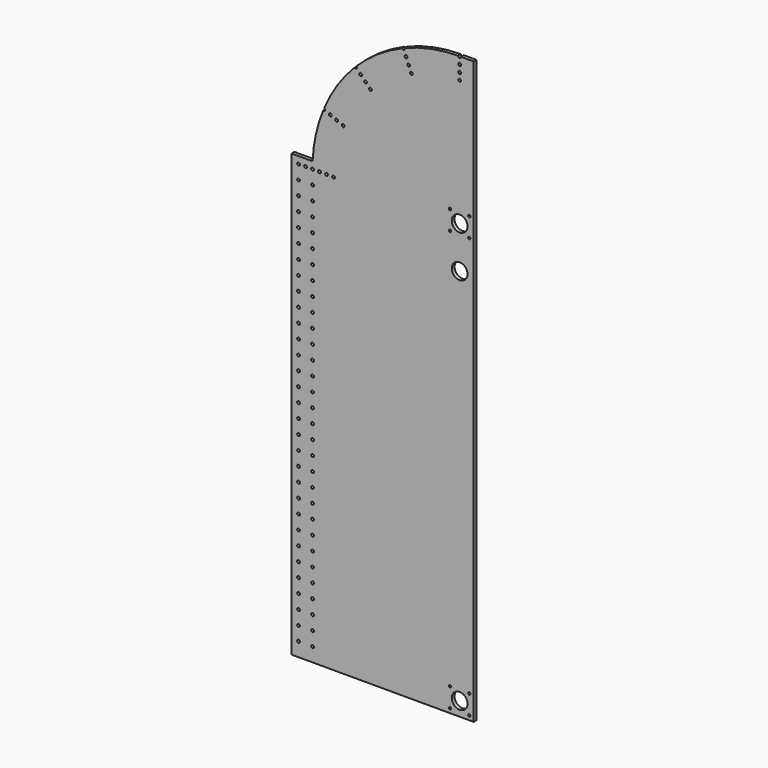
from build123d import *

# Parameters (mm, degrees)
F0_R     = 14.2875
F1_DEPTH = 6.35
F2_R     = 2.5527
F3_DEPTH = 25.4
F4_R     = 2.159
F5_DEPTH = 25.4
F7_D     = 5.1054
F9_DEPTH = 25.4


# Not quite as in the source:
# - a feature names something its author has since deleted; it is built from what else it names


with BuildPart() as f1:
    # F0 (on Front) → F1 (new body)
    with BuildSketch(Plane.XZ):
        Polygon((25.4, -787.4), (25.4, 0), (25.4, 304.8), (-304.8, 304.8), (-304.8, 0), (-304.8, -787.4), align=None)
        with Locations((0, -762)):
            Circle(F0_R, mode=Mode.SUBTRACT)
        with Locations((0, -76.2)):
            Circle(F0_R, mode=Mode.SUBTRACT)
        Circle(F0_R, mode=Mode.SUBTRACT)
    extrude(amount=F1_DEPTH)

    # F2 (on face) → F3 (cut)
    with BuildSketch(Plane.XZ.offset(6.35)):
        with Locations((-292.1, -25.4)):
            Circle(F2_R)
        with Locations((-292.1, -50.8)):
            Circle(F2_R)
        with Locations((-266.7, -50.8)):
            Circle(F2_R)
        with Locations((-266.7, -25.4)):
            Circle(F2_R)
        with Locations((-266.7, 0)):
            Circle(F2_R)
        with Locations((-292.1, 0)):
            Circle(F2_R)
        with Locations((-292.1, -76.2)):
            Circle(F2_R)
        with Locations((-266.7, -76.2)):
            Circle(F2_R)
        with Locations((-292.1, -101.6)):
            Circle(F2_R)
        with Locations((-266.7, -101.6)):
            Circle(F2_R)
        with Locations((-266.7, -127)):
            Circle(F2_R)
        with Locations((-292.1, -127)):
            Circle(F2_R)
        with Locations((-292.1, -152.4)):
            Circle(F2_R)
        with Locations((-266.7, -152.4)):
            Circle(F2_R)
        with Locations((-292.1, -177.8)):
            Circle(F2_R)
        with Locations((-266.7, -177.8)):
            Circle(F2_R)
        with Locations((-266.7, -203.2)):
            Circle(F2_R)
        with Locations((-292.1, -203.2)):
            Circle(F2_R)
        with Locations((-292.1, -228.6)):
            Circle(F2_R)
        with Locations((-266.7, -228.6)):
            Circle(F2_R)
        with Locations((-292.1, -254)):
            Circle(F2_R)
        with Locations((-266.7, -254)):
            Circle(F2_R)
        with Locations((-266.7, -279.4)):
            Circle(F2_R)
        with Locations((-292.1, -279.4)):
            Circle(F2_R)
        with Locations((-292.1, -304.8)):
            Circle(F2_R)
        with Locations((-266.7, -304.8)):
            Circle(F2_R)
        with Locations((-266.7, -330.2)):
            Circle(F2_R)
        with Locations((-292.1, -330.2)):
            Circle(F2_R)
        with Locations((-292.1, -355.6)):
            Circle(F2_R)
        with Locations((-266.7, -355.6)):
            Circle(F2_R)
        with Locations((-266.7, -381)):
            Circle(F2_R)
        with Locations((-292.1, -381)):
            Circle(F2_R)
        with Locations((-266.7, -406.4)):
            Circle(F2_R)
        with Locations((-292.1, -406.4)):
            Circle(F2_R)
        with Locations((-292.1, -431.8)):
            Circle(F2_R)
        with Locations((-266.7, -431.8)):
            Circle(F2_R)
        with Locations((-266.7, -457.2)):
            Circle(F2_R)
        with Locations((-292.1, -457.2)):
            Circle(F2_R)
        with Locations((-266.7, -482.6)):
            Circle(F2_R)
        with Locations((-292.1, -482.6)):
            Circle(F2_R)
        with Locations((-292.1, -508)):
            Circle(F2_R)
        with Locations((-266.7, -508)):
            Circle(F2_R)
        with Locations((-266.7, -533.4)):
            Circle(F2_R)
        with Locations((-292.1, -533.4)):
            Circle(F2_R)
        with Locations((-266.7, -558.8)):
            Circle(F2_R)
        with Locations((-292.1, -558.8)):
            Circle(F2_R)
        with Locations((-292.1, -584.2)):
            Circle(F2_R)
        with Locations((-266.7, -584.2)):
            Circle(F2_R)
        with Locations((-266.7, -609.6)):
            Circle(F2_R)
        with Locations((-292.1, -609.6)):
            Circle(F2_R)
        with Locations((-266.7, -635)):
            Circle(F2_R)
        with Locations((-292.1, -635)):
            Circle(F2_R)
        with Locations((-292.1, -660.4)):
            Circle(F2_R)
        with Locations((-266.7, -660.4)):
            Circle(F2_R)
        with Locations((-266.7, -685.8)):
            Circle(F2_R)
        with Locations((-292.1, -685.8)):
            Circle(F2_R)
        with Locations((-266.7, -711.2)):
            Circle(F2_R)
        with Locations((-292.1, -711.2)):
            Circle(F2_R)
        with Locations((-292.1, -736.6)):
            Circle(F2_R)
        with Locations((-266.7, -736.6)):
            Circle(F2_R)
        with Locations((-266.7, -762)):
            Circle(F2_R)
        with Locations((-292.1, -762)):
            Circle(F2_R)
    extrude(amount=-F3_DEPTH, mode=Mode.SUBTRACT)

    # F4 (on face) → F5 (cut)
    with BuildSketch(Plane.XZ.offset(6.35)):
        with Locations((-17.5, -744.5)):
            Circle(F4_R)
        with Locations((17.5, -744.5)):
            Circle(F4_R)
        with Locations((17.5, -779.5)):
            Circle(F4_R)
        with Locations((-17.5, -779.5)):
            Circle(F4_R)
        with Locations((17.5, -17.5)):
            Circle(F4_R)
        with Locations((17.5, 17.5)):
            Circle(F4_R)
        with Locations((-17.5, 17.5)):
            Circle(F4_R)
        with Locations((-17.5, -17.5)):
            Circle(F4_R)
    extrude(amount=-F5_DEPTH, mode=Mode.SUBTRACT)

    # F7 (through all)
    with Locations(Plane.XZ.offset(6.35)):
        with Locations((-87.4814326387, 211.1988611321), (-92.3415122297, 222.932131195), (-97.2015918207, 234.6654012579), (-102.0616714118, 246.3986713208), (-106.9217510028, 258.1319413837), (0, 266.7), (0, 254), (0, 241.3), (0, 228.6), (0, 279.4), (-266.7, 0), (-254, 0), (-279.4, 0), (-258.1319413837, 106.9217510028), (-246.3986713208, 102.0616714118), (-234.6654012579, 97.2015918207), (-241.3, 0), (-228.6, 0), (-222.932131195, 92.3415122297), (-161.6446101792, 161.6446101792), (-170.6248663003, 170.6248663003), (-188.5853785425, 188.5853785425), (-179.6051224214, 179.6051224214), (-211.1988611321, 87.4814326387), (-197.5656346635, 197.5656346635)):
            Hole(F7_D / 2)

    # F8 (on face) → F9 (cut)
    with BuildSketch(Plane.XZ.offset(6.35)):
        with BuildLine():
            Line((-304.8, 304.8), (-304.8, 12.7))
            Line((-304.8, 12.7), (-266.7, 12.7))
            ThreePointArc((-266.7, 12.7), (-184.2542427414, 193.2370410449), (0, 267.0022097287))
            Line((0, 267.0022097287), (25.4, 267.0022097287))
            Line((25.4, 267.0022097287), (25.4, 304.8))
            Line((25.4, 304.8), (-304.8, 304.8))
        make_face()
    extrude(amount=-F9_DEPTH, mode=Mode.SUBTRACT)


solid = f1.part
